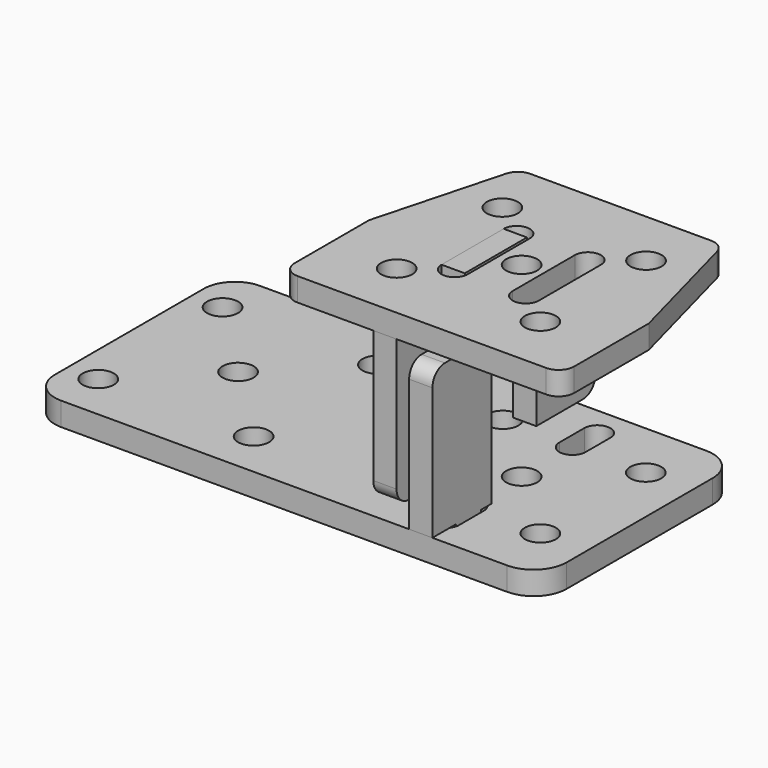
from build123d import *

# Parameters (mm, degrees)
F0_R      = 6.35
F1_DEPTH  = 9.525
F3_DEPTH  = 25.4
F5_R      = 6.35
F6_DEPTH  = 9.525
F8_DEPTH  = 25.4
F10_DEPTH = 9.525
F12_DEPTH = 9.525


# Not quite as in the source:
# - ends of sketch curves that miss each other by under 0.0002 mm in the source are joined


with BuildPart() as f1:
    # F0 (on Top) → F1 (new body)
    with BuildSketch(Plane.XY):
        with BuildLine():
            ThreePointArc((-97.5487, -38.1), (-93.8289561211, -47.0802561211), (-84.8487, -50.8))
            Line((-84.8487, -50.8), (97.5487, -50.8))
            ThreePointArc((97.5487, -50.8), (107.0947122567, -46.8459122567), (111.0488, -37.2999))
            Line((111.0488, -37.2999), (111.0488, 37.2999))
            ThreePointArc((111.0488, 37.2999), (107.0947122567, 46.8459122567), (97.5487, 50.8))
            Line((97.5487, 50.8), (-84.8487, 50.8))
            ThreePointArc((-84.8487, 50.8), (-93.8289561211, 47.0802561211), (-97.5487, 38.1))
            Line((-97.5487, 38.1), (-97.5487, -38.1))
        make_face()
        with Locations((-84.8487, -31.75)):
            Circle(F0_R, mode=Mode.SUBTRACT)
        with Locations((-21.3487, -31.75)):
            Circle(F0_R, mode=Mode.SUBTRACT)
        with Locations((33.5788, -26.924)):
            Circle(F0_R, mode=Mode.SUBTRACT)
        with Locations((91.9988, -26.924)):
            Circle(F0_R, mode=Mode.SUBTRACT)
        with Locations((-53.0987, 0)):
            Circle(F0_R, mode=Mode.SUBTRACT)
        with Locations((62.7888, 0)):
            Circle(F0_R, mode=Mode.SUBTRACT)
        with Locations((33.5788, 26.924)):
            Circle(F0_R, mode=Mode.SUBTRACT)
        with Locations((91.9988, 26.924)):
            Circle(F0_R, mode=Mode.SUBTRACT)
        with Locations((-84.8487, 31.75)):
            Circle(F0_R, mode=Mode.SUBTRACT)
        with Locations((-21.3487, 31.75)):
            Circle(F0_R, mode=Mode.SUBTRACT)
    extrude(amount=F1_DEPTH)

    # F2 (on face) → F3 (cut)
    with BuildSketch(Plane.XY.offset(9.525)):
        with BuildLine():
            ThreePointArc((57.4548, 25.9715), (62.7888, 20.6375), (68.1228, 25.9715))
            Line((68.1228, 25.9715), (68.1228, 38.6715))
            ThreePointArc((68.1228, 38.6715), (62.7888, 44.0055), (57.4548, 38.6715))
            Line((57.4548, 38.6715), (57.4548, 25.9715))
        make_face()
        with BuildLine():
            ThreePointArc((57.4548, -38.6715), (62.7888, -44.0055), (68.1228, -38.6715))
            Line((68.1228, -38.6715), (68.1228, -25.9715))
            ThreePointArc((68.1228, -25.9715), (62.7888, -20.6375), (57.4548, -25.9715))
            Line((57.4548, -25.9715), (57.4548, -38.6715))
        make_face()
    extrude(amount=-F3_DEPTH, mode=Mode.SUBTRACT)


with BuildPart() as f6:
    # F5 (on offset) → F6 (new body)
    with BuildSketch(Plane.XY.offset(76.2)):
        with BuildLine():
            Line((99.5942382, 50.8634627833), (25.6658618, 50.8634627833))
            ThreePointArc((25.6658618, 50.8634627833), (21.8002302398, 49.5512591905), (19.5322350958, 46.1569722763))
            Line((19.5322350958, 46.1569722763), (5.48005, -6.2865))
            Line((5.48005, -6.2865), (5.48005, -44.3865))
            ThreePointArc((5.48005, -44.3865), (7.3399219395, -48.8766280605), (11.83005, -50.7365))
            Line((11.83005, -50.7365), (113.43005, -50.7365372167))
            ThreePointArc((113.43005, -50.7365372167), (117.9201780605, -48.8766652773), (119.78005, -44.3865372167))
            Line((119.78005, -44.3865372167), (119.78005, -6.2865))
            Line((119.78005, -6.2865), (105.7278649042, 46.1569722763))
            ThreePointArc((105.7278649042, 46.1569722763), (103.4598697602, 49.5512591905), (99.5942382, 50.8634627833))
        make_face()
        with Locations((33.2613, -26.924)):
            Circle(F5_R, mode=Mode.SUBTRACT)
        with Locations((91.9988, -26.924)):
            Circle(F5_R, mode=Mode.SUBTRACT)
        with Locations((62.7888, 0)):
            Circle(F5_R, mode=Mode.SUBTRACT)
        with Locations((33.2613, 27.051)):
            Circle(F5_R, mode=Mode.SUBTRACT)
        with Locations((91.9988, 27.051)):
            Circle(F5_R, mode=Mode.SUBTRACT)
    extrude(amount=F6_DEPTH)

    # F7 (on face) → F8 (cut)
    with BuildSketch(Plane(origin=(0, 0, 76.2), x_dir=(1, 0, 0), z_dir=(0, 0, -1))):
        with BuildLine():
            ThreePointArc((71.8439, -15.875), (77.1779, -21.209), (82.5119, -15.875))
            Line((82.5119, -15.875), (82.5119, 15.875))
            ThreePointArc((82.5119, 15.875), (77.1779, 21.209), (71.8439, 15.875))
            Line((71.8439, 15.875), (71.8439, -15.875))
        make_face()
        with BuildLine():
            ThreePointArc((42.7482, -15.875), (48.0822, -21.209), (53.4162, -15.875))
            Line((53.4162, -15.875), (53.4162, 15.875))
            ThreePointArc((53.4162, 15.875), (48.0822, 21.209), (42.7482, 15.875))
            Line((42.7482, 15.875), (42.7482, -15.875))
        make_face()
    extrude(amount=-F8_DEPTH, mode=Mode.SUBTRACT)


with BuildPart() as f10:
    # F9 (on face) → F10 (new body)
    with BuildSketch(Plane.YZ.offset(42.7482)):
        with BuildLine():
            Line((15.875, 76.2), (15.875, 85.725))
            Line((15.875, 85.725), (-15.875, 85.725))
            Line((-15.875, 85.725), (-15.875, 76.2))
            Line((-15.875, 76.2), (-50.7365372167, 76.2))
            Line((-50.7365372167, 76.2), (-50.7365372167, 22.225))
            ThreePointArc((-50.7365372167, 22.225), (-48.8766652773, 17.7348719395), (-44.3865372167, 15.875))
            Line((-44.3865372167, 15.875), (-20.6375, 15.875))
            Line((-20.6375, 15.875), (-20.6375, 52.8731126447))
            ThreePointArc((-20.6375, 52.8731126447), (0, 54.4606126447), (20.6375, 52.8731126447))
            Line((20.6375, 52.8731126447), (20.6375, 15.875))
            Line((20.6375, 15.875), (44.5134627833, 15.875))
            ThreePointArc((44.5134627833, 15.875), (49.0035908438, 17.7348719395), (50.8634627833, 22.225))
            Line((50.8634627833, 22.225), (50.8634627833, 76.2))
            Line((50.8634627833, 76.2), (15.875, 76.2))
        make_face()
    extrude(amount=F10_DEPTH)


with BuildPart() as f12:
    # F11 (on face) → F12 (new body)
    with BuildSketch(Plane.YZ.offset(57.4548)):
        with BuildLine():
            Line((-38.6715, 0), (-25.9715, 0))
            Line((-25.9715, 0), (-25.9715, 9.525))
            Line((-25.9715, 9.525), (-20.6375, 9.525))
            Line((-20.6375, 9.525), (-20.6375, 63.5))
            ThreePointArc((-20.6375, 63.5), (-22.4973719395, 67.9901280605), (-26.9875, 69.85))
            Line((-26.9875, 69.85), (-44.45, 69.85))
            ThreePointArc((-44.45, 69.85), (-48.9401280605, 67.9901280605), (-50.8, 63.5))
            Line((-50.8, 63.5), (-50.8, 9.525))
            Line((-50.8, 9.525), (-38.6715, 9.525))
            Line((-38.6715, 9.525), (-38.6715, 0))
        make_face()
    extrude(amount=F12_DEPTH)


solid = Compound([f1.part, f6.part, f10.part, f12.part])
